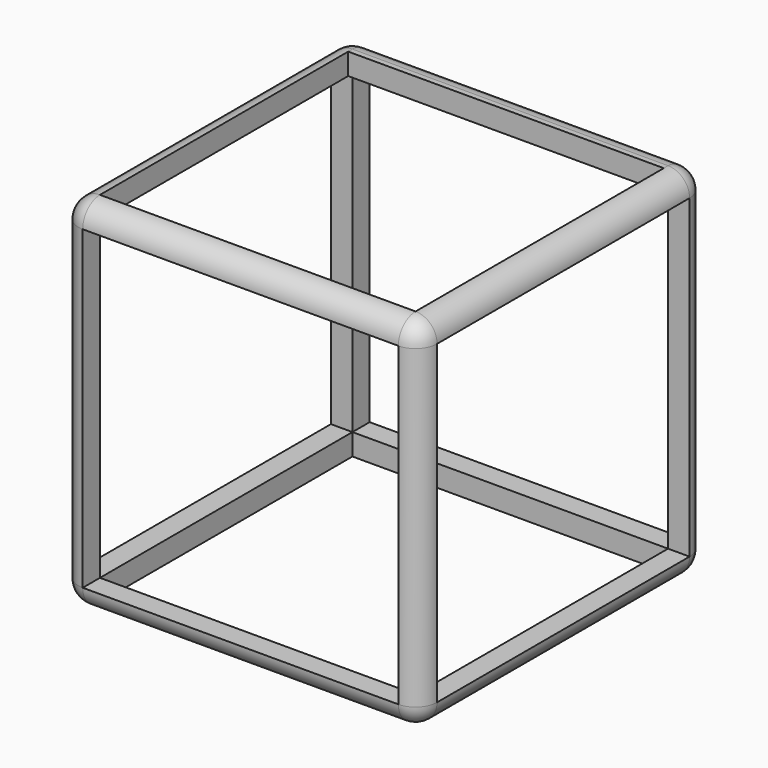
from build123d import *

# Parameters (mm, degrees)
F0_W      = 50.8
F0_H      = 50.8
F0_W_2    = 44.704000783
F0_H_2    = 44.704000783
F9_DEPTH  = 3.048
F1_W      = 50.8
F1_H      = 50.8
F1_W_2    = 44.704000783
F1_H_2    = 44.704000783
F10_DEPTH = 3.048
F2_W      = 50.8
F2_H      = 50.8
F2_W_2    = 44.704000783
F2_H_2    = 44.704000783
F11_DEPTH = 3.048
F6_W      = 50.8
F6_H      = 50.8
F6_W_2    = 44.704000783
F6_H_2    = 44.704000783
F12_DEPTH = 3.048
F7_W      = 50.8
F7_H      = 50.8
F7_W_2    = 44.704000783
F7_H_2    = 44.704000783
F13_DEPTH = 3.048
F8_W      = 50.8
F8_H      = 50.0440469261
F8_W_2    = 44.7040001482
F8_H_2    = 43.9480470743
F14_DEPTH = 3.048
F15_R     = 3.04799


# Not quite as in the source:
# - a fillet or chamfer is up to 0.001 mm smaller than in the source, because OpenCascade refuses the exact size


with BuildPart() as f9:
    # F0 (on Top) → F9 (new body)
    with BuildSketch(Plane.XY):
        with Locations((25.4, 25.4)):
            Rectangle(F0_W, F0_H)
        with Locations((25.4, 25.4)):
            Rectangle(F0_W_2, F0_H_2, mode=Mode.SUBTRACT)
    extrude(amount=F9_DEPTH)

    # F1 (on Front) → F10 (join)
    with BuildSketch(Plane.XZ):
        with Locations((25.4, 25.4)):
            Rectangle(F1_W, F1_H)
        with Locations((25.4, 25.4)):
            Rectangle(F1_W_2, F1_H_2, mode=Mode.SUBTRACT)
    extrude(amount=-F10_DEPTH)

    # F2 (on Right) → F11 (join)
    with BuildSketch(Plane.YZ):
        with Locations((25.4, 25.4)):
            Rectangle(F2_W, F2_H)
        with Locations((25.4, 25.4)):
            Rectangle(F2_W_2, F2_H_2, mode=Mode.SUBTRACT)
    extrude(amount=F11_DEPTH)

    # F6 (on offset) → F12 (join)
    with BuildSketch(Plane.YZ.offset(50.8)):
        with Locations((25.4, 25.4)):
            Rectangle(F6_W, F6_H)
        with Locations((25.4, 25.4)):
            Rectangle(F6_W_2, F6_H_2, mode=Mode.SUBTRACT)
    extrude(amount=-F12_DEPTH)

    # F7 (on offset) → F13 (join)
    with BuildSketch(Plane.XZ.offset(-50.8)):
        with Locations((25.4, 25.4)):
            Rectangle(F7_W, F7_H)
        with Locations((25.4, 25.4)):
            Rectangle(F7_W_2, F7_H_2, mode=Mode.SUBTRACT)
    extrude(amount=F13_DEPTH)

    # F8 (on offset) → F14 (join)
    with BuildSketch(Plane.XY.offset(50.8)):
        with Locations((25.4, 25.022023463)):
            Rectangle(F8_W, F8_H)
        with Locations((25.4, 25.022023463)):
            Rectangle(F8_W_2, F8_H_2, mode=Mode.SUBTRACT)
    extrude(amount=-F14_DEPTH)

    # F15 (radius 3.048 in the source; OpenCascade refuses exactly that, so slightly less here)
    f15_edges = [f9.edges().sort_by_distance(p)[0] for p in [
        (50.8, 50.8, 25.4),
        (25.4, 50.8, 0),
        (50.8, 25.4, 0),
        (25.4, 0, 0),
        (50.8, 0, 25.4),
        (50.8, 25.4, 50.8),
        (25.4, 50.8, 50.8),
        (25.4, 0, 50.8),
        (0, 25.4, 50.8),
        (0, 50.8, 25.4),
        (0, 25.4, 0),
        (0, 0, 25.4),
    ]]
    fillet(f15_edges, radius=F15_R)


solid = f9.part
